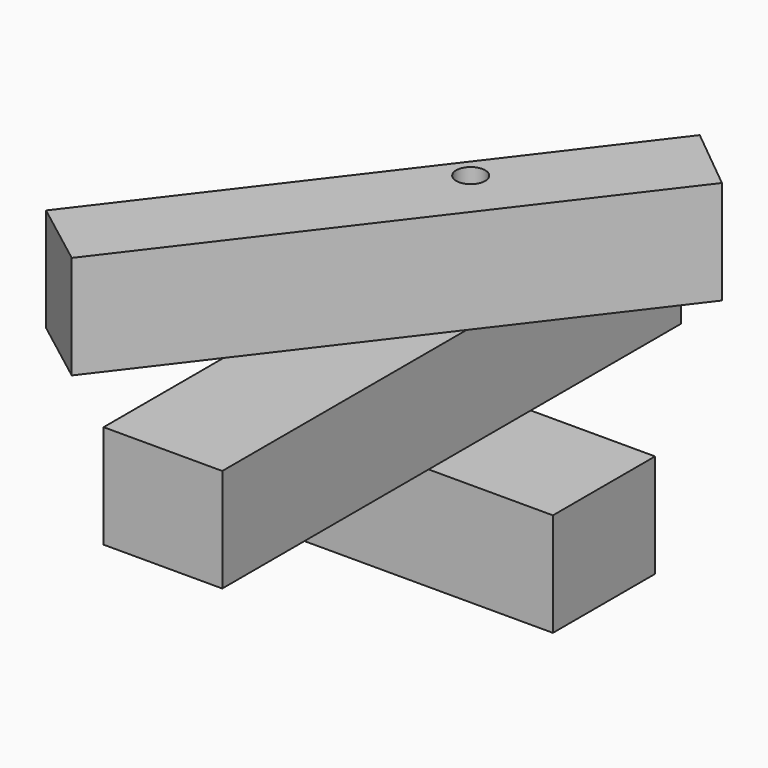
from build123d import *

# Parameters (mm, degrees)
F0_W     = 81.6161185503
F0_H     = 30.8448886499
F1_DEPTH = 25
F2_W     = 28.6611793563
F2_H     = 138.4778022766
F2_H_2   = 45.3190533444
F3_DEPTH = 25
F5_DEPTH = 25
F7_D     = 7


# Not quite as in the source:
# - a feature names something its author has since deleted; it is built from what else it names


with BuildPart() as f1:
    # F0 (on Top) → F1 (new body)
    with BuildSketch(Plane.XY):
        with Locations((6.8240910769, -1.094697509)):
            Rectangle(F0_W, F0_H)
    extrude(amount=F1_DEPTH)


with BuildPart() as f3:
    # F2 (on face) → F3 (new body)
    with BuildSketch(Plane.XY.offset(25)):
        with Locations((3.2755625434, -9.5921009779)):
            Rectangle(F2_W, F2_H)
        with Locations((3.2755625434, 36.9872734882)):
            Rectangle(F2_W, F2_H_2)
    extrude(amount=F3_DEPTH)


with BuildPart() as f5:
    # F4 (on face) → F5 (new body)
    with BuildSketch(Plane.XY.offset(50)):
        Polygon((47.707793434, 34.4260234633), (32.224177393, 47.0853138974), (-44.8405611611, -53.9763291491), (-28.9460210758, -66.0967394174), align=None)
    extrude(amount=F5_DEPTH)

    # F7 (through all)
    with Locations(Plane.XY.offset(75)):
        with Locations((8.8179567829, 7.1794758551)):
            Hole(F7_D / 2)


solid = Compound([f1.part, f3.part, f5.part])
